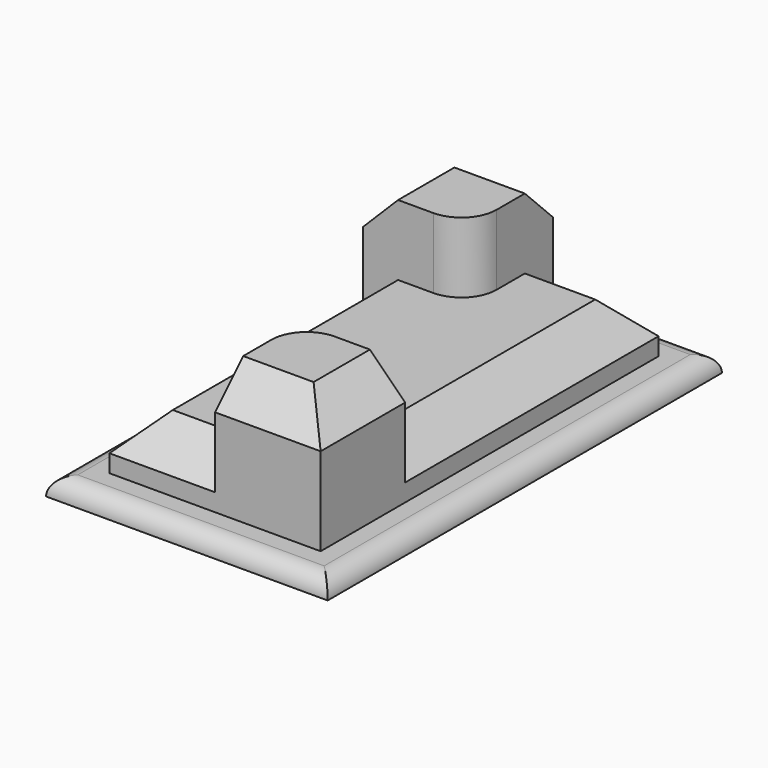
from build123d import *

# Parameters (mm, degrees)
F1_DEPTH = 25.4
F2_DEPTH = 50.8
F0_W     = 101.6
F0_H     = 177.8
F3_DEPTH = 6.35
F4_R     = 6.34999
F5_SIZE  = 12.7
F6_SIZE  = 12.7


# Not quite as in the source:
# - a fillet or chamfer is up to 0.001 mm smaller than in the source, because OpenCascade refuses the exact size
# - a length typed as a fraction of an inch, garbled in the dataset ("3 / 203.2 mm" for 3/8 in), is restored


with BuildPart() as f1:
    # F0 (on Top) → F1 (new body)
    with BuildSketch(Plane.XY):
        with BuildLine():
            Line((44.7456893295, 103.9061718148), (6.6456893295, 103.9061718148))
            Line((6.6456893295, 103.9061718148), (6.6456893295, 78.5061718148))
            ThreePointArc((6.6456893295, 78.5061718148), (2.9259454506, 69.5259156938), (-6.0543106705, 65.8061718148))
            Line((-6.0543106705, 65.8061718148), (-31.4543106705, 65.8061718148))
            Line((-31.4543106705, 65.8061718148), (-31.4543106705, -48.4938281852))
            Line((-31.4543106705, -48.4938281852), (6.6456893295, -48.4938281852))
            Line((6.6456893295, -48.4938281852), (6.6456893295, -23.0938281852))
            ThreePointArc((6.6456893295, -23.0938281852), (10.3654332084, -14.1135720641), (19.3456893295, -10.3938281852))
            Line((19.3456893295, -10.3938281852), (44.7456893295, -10.3938281852))
            Line((44.7456893295, -10.3938281852), (44.7456893295, 103.9061718148))
        make_face()
    extrude(amount=F1_DEPTH)

    # F0 (on Top) → F2 (join)
    with BuildSketch(Plane.XY):
        with BuildLine():
            Line((6.6456893295, 103.9061718148), (-31.4543106705, 103.9061718148))
            Line((-31.4543106705, 103.9061718148), (-31.4543106705, 65.8061718148))
            Line((-31.4543106705, 65.8061718148), (-6.0543106705, 65.8061718148))
            ThreePointArc((-6.0543106705, 65.8061718148), (2.9259454506, 69.5259156938), (6.6456893295, 78.5061718148))
            Line((6.6456893295, 78.5061718148), (6.6456893295, 103.9061718148))
        make_face()
        with BuildLine():
            Line((44.7456893295, -48.4938281852), (44.7456893295, -10.3938281852))
            Line((44.7456893295, -10.3938281852), (19.3456893295, -10.3938281852))
            ThreePointArc((19.3456893295, -10.3938281852), (10.3654332084, -14.1135720641), (6.6456893295, -23.0938281852))
            Line((6.6456893295, -23.0938281852), (6.6456893295, -48.4938281852))
            Line((6.6456893295, -48.4938281852), (44.7456893295, -48.4938281852))
        make_face()
    extrude(amount=F2_DEPTH)

    # F0 (on Top) → F3 (join)
    with BuildSketch(Plane.XY):
        with Locations((6.6456893295, 27.7061718148)):
            Rectangle(F0_W, F0_H)
        Polygon((-31.4543106705, 65.8061718148), (-31.4543106705, 103.9061718148), (6.6456893295, 103.9061718148), (44.7456893295, 103.9061718148), (44.7456893295, -10.3938281852), (44.7456893295, -48.4938281852), (6.6456893295, -48.4938281852), (-31.4543106705, -48.4938281852), align=None, mode=Mode.SUBTRACT)
    extrude(amount=F3_DEPTH)

    # F4 (radius 6.35 in the source; OpenCascade refuses exactly that, so slightly less here)
    f4_edges = [f1.edges().sort_by_distance(p)[0] for p in [
        (6.645689, -61.193828, 6.35),
        (-44.154311, 27.706172, 6.35),
        (6.645689, 116.606172, 6.35),
        (57.445689, 27.706172, 6.35),
    ]]
    fillet(f4_edges, radius=F4_R)

    # F5
    f5_edges = [f1.edges().sort_by_distance(p)[0] for p in [
        (-12.404311, -48.493828, 25.4),
        (-31.454311, 8.656172, 25.4),
        (44.745689, 46.756172, 25.4),
        (25.695689, 103.906172, 25.4),
    ]]
    chamfer(f5_edges, length=F5_SIZE)

    # F6
    f6_edges = [f1.edges().sort_by_distance(p)[0] for p in [
        (44.745689, -29.443828, 50.8),
        (25.695689, -48.493828, 50.8),
        (-31.454311, 84.856172, 50.8),
        (-12.404311, 103.906172, 50.8),
    ]]
    chamfer(f6_edges, length=F6_SIZE)


solid = f1.part
